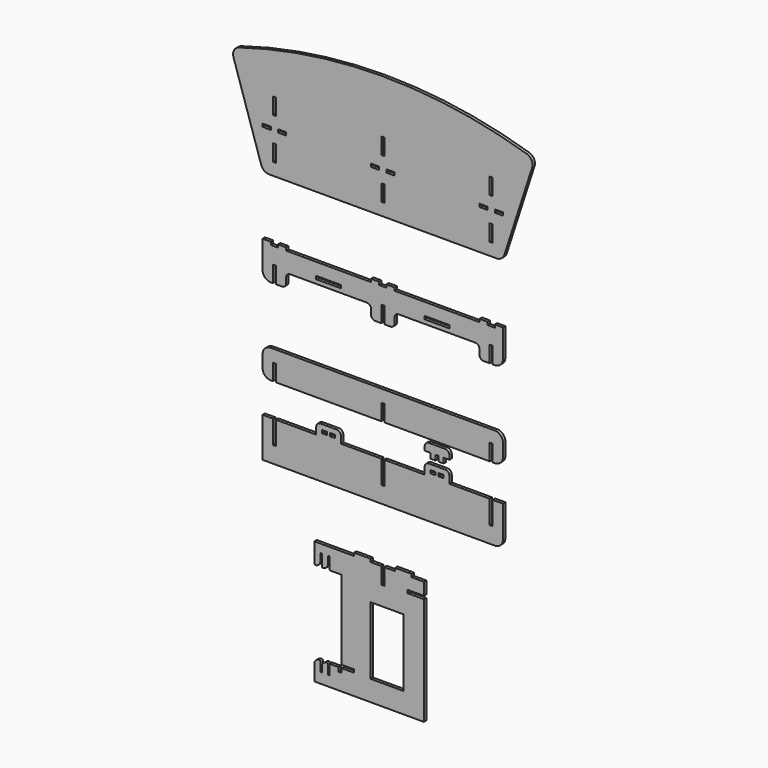
from build123d import *

# Parameters (mm, degrees)
F0_W     = 203.2
F0_H     = 417.195
F1_DEPTH = 18.542
F0_W_2   = 152.4
F0_H_2   = 18.542
F0_W_3   = 50.8
F0_H_3   = 18.034
F0_W_4   = 18.542
F0_H_4   = 101.6
F0_W_5   = 31.75
F0_H_5   = 31.75


# Not quite as in the source:
# - a feature names something its author has since deleted; it is built from what else it names


with BuildPart() as f1:
    # F0 (on Front) → F1 (new body)
    with BuildSketch(Plane.XZ):
        with BuildLine():
            Line((-177.8, 381), (-254, 381))
            Line((-254, 381), (-423.3333333333, 381))
            Line((-423.3333333333, 381), (-423.3333333333, 260.35))
            ThreePointArc((-423.3333333333, 260.35), (-421.4734613939, 255.8598719395), (-416.9833333333, 254))
            ThreePointArc((-416.9833333333, 254), (-394.5326930307, 263.2993596973), (-385.2333333333, 285.75))
            Line((-385.2333333333, 285.75), (-385.2333333333, 317.5))
            Line((-385.2333333333, 317.5), (-385.2333333333, 330.2))
            Line((-385.2333333333, 330.2), (-376.3433333333, 330.2))
            Line((-376.3433333333, 330.2), (-376.3433333333, 317.5))
            Line((-376.3433333333, 317.5), (-376.3433333333, 260.35))
            ThreePointArc((-376.3433333333, 260.35), (-374.4834613939, 255.8598719395), (-369.9933333333, 254))
            ThreePointArc((-369.9933333333, 254), (-347.5426930307, 263.2993596973), (-338.2433333333, 285.75))
            Line((-338.2433333333, 285.75), (-338.2433333333, 317.5))
            Line((-338.2433333333, 317.5), (-338.2433333333, 330.2))
            Line((-338.2433333333, 330.2), (-329.3533333333, 330.2))
            Line((-329.3533333333, 330.2), (-329.3533333333, 317.5))
            Line((-329.3533333333, 317.5), (-329.3533333333, 260.35))
            ThreePointArc((-329.3533333333, 260.35), (-327.4934613939, 255.8598719395), (-323.0033333333, 254))
            Line((-323.0033333333, 254), (-254, 254))
            Line((-254, 254), (-254, -235.458))
            Line((-254, -235.458), (-177.8, -235.458))
            Line((-177.8, -235.458), (-177.8, -254))
            Line((-177.8, -254), (-254, -254))
            Line((-254, -254), (-254, -279.4))
            Line((-254, -279.4), (-272.542, -279.4))
            Line((-272.542, -279.4), (-272.542, -254))
            Line((-272.542, -254), (-329.3533333333, -254))
            Line((-329.3533333333, -254), (-329.3533333333, -317.5))
            Line((-329.3533333333, -317.5), (-338.2433333333, -317.5))
            Line((-338.2433333333, -317.5), (-338.2433333333, -260.35))
            ThreePointArc((-338.2433333333, -260.35), (-340.1032052728, -255.8598719395), (-344.5933333333, -254))
            ThreePointArc((-344.5933333333, -254), (-367.043973636, -263.2993596973), (-376.3433333333, -285.75))
            Line((-376.3433333333, -285.75), (-376.3433333333, -317.5))
            Line((-376.3433333333, -317.5), (-385.2333333333, -317.5))
            Line((-385.2333333333, -317.5), (-385.2333333333, -260.35))
            ThreePointArc((-385.2333333333, -260.35), (-387.0932052728, -255.8598719395), (-391.5833333333, -254))
            ThreePointArc((-391.5833333333, -254), (-414.033973636, -263.2993596973), (-423.3333333333, -285.75))
            Line((-423.3333333333, -285.75), (-423.3333333333, -381))
            Line((-423.3333333333, -381), (-254, -381))
            Line((-254, -381), (254, -381))
            Line((254, -381), (254, 286.258))
            Line((254, 286.258), (152.4, 286.258))
            Line((152.4, 286.258), (152.4, 304.8))
            Line((152.4, 304.8), (254, 304.8))
            Line((254, 304.8), (254, 381))
            Line((254, 381), (177.8, 381))
            Line((177.8, 381), (177.8, 399.1356))
            Line((177.8, 399.1356), (76.2, 399.1356))
            Line((76.2, 399.1356), (76.2, 381))
            Line((76.2, 381), (9.0678, 381))
            Line((9.0678, 381), (9.0678, 279.4))
            Line((9.0678, 279.4), (-9.0678, 279.4))
            Line((-9.0678, 279.4), (-9.0678, 381))
            Line((-9.0678, 381), (-76.2, 381))
            Line((-76.2, 381), (-76.2, 399.1356))
            Line((-76.2, 399.1356), (-177.8, 399.1356))
            Line((-177.8, 399.1356), (-177.8, 381))
        make_face()
        with Locations((25.4, -45.4025)):
            Rectangle(F0_W, F0_H, mode=Mode.SUBTRACT)
    extrude(amount=F1_DEPTH)


with BuildPart() as f1b:
    # F0 (on Front) → F1, piece 2 (new body)
    with BuildSketch(Plane.XZ):
        with BuildLine():
            Line((691.945207411, 1346.2), (-691.945207411, 1346.2))
            ThreePointArc((-691.945207411, 1346.2), (-727.8662318953, 1331.3210244843), (-742.745207411, 1295.4))
            Line((-742.745207411, 1295.4), (-742.745207411, 1219.2))
            ThreePointArc((-742.745207411, 1219.2), (-727.8662318953, 1183.2789755157), (-691.945207411, 1168.4))
            Line((-691.945207411, 1168.4), (-679.245207411, 1168.4))
            Line((-679.245207411, 1168.4), (-679.245207411, 1270))
            Line((-679.245207411, 1270), (-660.703207411, 1270))
            Line((-660.703207411, 1270), (-660.703207411, 1168.4))
            Line((-660.703207411, 1168.4), (-9.271, 1168.4))
            Line((-9.271, 1168.4), (-9.271, 1270))
            Line((-9.271, 1270), (9.271, 1270))
            Line((9.271, 1270), (9.271, 1168.4))
            Line((9.271, 1168.4), (660.703207411, 1168.4))
            Line((660.703207411, 1168.4), (660.703207411, 1270))
            Line((660.703207411, 1270), (679.245207411, 1270))
            Line((679.245207411, 1270), (679.245207411, 1168.4))
            Line((679.245207411, 1168.4), (691.945207411, 1168.4))
            ThreePointArc((691.945207411, 1168.4), (727.8662318953, 1183.2789755157), (742.745207411, 1219.2))
            Line((742.745207411, 1219.2), (742.745207411, 1295.4))
            ThreePointArc((742.745207411, 1295.4), (727.8662318953, 1331.3210244843), (691.945207411, 1346.2))
        make_face()
    extrude(amount=F1_DEPTH)


with BuildPart() as f1c:
    # F0 (on Front) → F1, piece 3 (new body)
    with BuildSketch(Plane.XZ):
        with BuildLine():
            Line((-691.945207411, 1905), (-742.745207411, 1905))
            Line((-742.745207411, 1905), (-742.745207411, 1752.6))
            ThreePointArc((-742.745207411, 1752.6), (-727.8662318953, 1716.6789755157), (-691.945207411, 1701.8))
            Line((-691.945207411, 1701.8), (-679.245207411, 1701.8))
            Line((-679.245207411, 1701.8), (-679.245207411, 1803.4))
            Line((-679.245207411, 1803.4), (-660.703207411, 1803.4))
            Line((-660.703207411, 1803.4), (-660.703207411, 1701.8))
            Line((-660.703207411, 1701.8), (-622.603207411, 1701.8))
            ThreePointArc((-622.603207411, 1701.8), (-604.6426951688, 1709.2394877579), (-597.203207411, 1727.2))
            Line((-597.203207411, 1727.2), (-597.203207411, 1759.458))
            ThreePointArc((-597.203207411, 1759.458), (-589.7637196531, 1777.4185122421), (-571.803207411, 1784.858))
            Line((-571.803207411, 1784.858), (-98.171, 1784.858))
            ThreePointArc((-98.171, 1784.858), (-80.2104877579, 1777.4185122421), (-72.771, 1759.458))
            Line((-72.771, 1759.458), (-72.771, 1727.2))
            ThreePointArc((-72.771, 1727.2), (-65.3315122421, 1709.2394877579), (-47.371, 1701.8))
            Line((-47.371, 1701.8), (-9.271, 1701.8))
            Line((-9.271, 1701.8), (-9.271, 1803.4))
            Line((-9.271, 1803.4), (9.271, 1803.4))
            Line((9.271, 1803.4), (9.271, 1701.8))
            Line((9.271, 1701.8), (47.371, 1701.8))
            ThreePointArc((47.371, 1701.8), (65.3315122421, 1709.2394877579), (72.771, 1727.2))
            Line((72.771, 1727.2), (72.771, 1759.458))
            ThreePointArc((72.771, 1759.458), (80.2104877579, 1777.4185122421), (98.171, 1784.858))
            Line((98.171, 1784.858), (571.803207411, 1784.858))
            ThreePointArc((571.803207411, 1784.858), (589.7637196531, 1777.4185122421), (597.203207411, 1759.458))
            Line((597.203207411, 1759.458), (597.203207411, 1727.2))
            ThreePointArc((597.203207411, 1727.2), (604.6426951688, 1709.2394877579), (622.603207411, 1701.8))
            Line((622.603207411, 1701.8), (660.703207411, 1701.8))
            Line((660.703207411, 1701.8), (660.703207411, 1803.4))
            Line((660.703207411, 1803.4), (679.245207411, 1803.4))
            Line((679.245207411, 1803.4), (679.245207411, 1701.8))
            Line((679.245207411, 1701.8), (691.945207411, 1701.8))
            ThreePointArc((691.945207411, 1701.8), (727.8662318953, 1716.6789755157), (742.745207411, 1752.6))
            Line((742.745207411, 1752.6), (742.745207411, 1905))
            Line((742.745207411, 1905), (691.945207411, 1905))
            Line((691.945207411, 1905), (648.003207411, 1905))
            Line((648.003207411, 1905), (597.203207411, 1905))
            Line((597.203207411, 1905), (72.771, 1905))
            Line((72.771, 1905), (21.971, 1905))
            Line((21.971, 1905), (-21.971, 1905))
            Line((-21.971, 1905), (-72.771, 1905))
            Line((-72.771, 1905), (-597.203207411, 1905))
            Line((-597.203207411, 1905), (-648.003207411, 1905))
            Line((-648.003207411, 1905), (-691.945207411, 1905))
        make_face()
        with Locations((-334.9871037055, 1819.529)):
            Rectangle(F0_W_2, F0_H_2, mode=Mode.SUBTRACT)
        with Locations((334.9871037055, 1819.529)):
            Rectangle(F0_W_2, F0_H_2, mode=Mode.SUBTRACT)
        with Locations((-717.345207411, 1914.017)):
            Rectangle(F0_W_3, F0_H_3)
        with Locations((-622.603207411, 1914.017)):
            Rectangle(F0_W_3, F0_H_3)
        with Locations((-47.371, 1914.017)):
            Rectangle(F0_W_3, F0_H_3)
        with Locations((47.371, 1914.017)):
            Rectangle(F0_W_3, F0_H_3)
        with Locations((622.603207411, 1914.017)):
            Rectangle(F0_W_3, F0_H_3)
        with Locations((717.345207411, 1914.017)):
            Rectangle(F0_W_3, F0_H_3)
    extrude(amount=F1_DEPTH)


with BuildPart() as f1d:
    # F0 (on Front) → F1, piece 4 (new body)
    with BuildSketch(Plane.XZ):
        with BuildLine():
            ThreePointArc((0, 3048), (-449.4470794405, 3014.6809653399), (-889.0679496829, 2915.452311537))
            ThreePointArc((-889.0679496829, 2915.452311537), (-919.2876316446, 2890.361765082), (-922.5828932993, 2851.2221949528))
            Line((-922.5828932993, 2851.2221949528), (-751.0685099201, 2321.1607552747))
            ThreePointArc((-751.0685099201, 2321.1607552747), (-732.6202645277, 2295.7201166503), (-702.7357671423, 2286))
            Line((-702.7357671423, 2286), (0, 2286))
            Line((0, 2286), (702.7357671423, 2286))
            ThreePointArc((702.7357671423, 2286), (732.6202645277, 2295.7201166503), (751.0685099201, 2321.1607552747))
            Line((751.0685099201, 2321.1607552747), (922.5828932993, 2851.2221949528))
            ThreePointArc((922.5828932993, 2851.2221949528), (919.2876316446, 2890.361765082), (889.0679496829, 2915.452311537))
            ThreePointArc((889.0679496829, 2915.452311537), (449.4470794405, 3014.6809653399), (0, 3048))
        make_face()
        with Locations((-717.345207411, 2540.2032)):
            Rectangle(F0_W_3, F0_H_2, mode=Mode.SUBTRACT)
        with Locations((-669.974207411, 2413)):
            Rectangle(F0_W_4, F0_H_4, mode=Mode.SUBTRACT)
        with Locations((-622.603207411, 2540.2032)):
            Rectangle(F0_W_3, F0_H_2, mode=Mode.SUBTRACT)
        with Locations((-669.974207411, 2667.4064)):
            Rectangle(F0_W_4, F0_H_4, mode=Mode.SUBTRACT)
        with Locations((-47.371, 2540.2032)):
            Rectangle(F0_W_3, F0_H_2, mode=Mode.SUBTRACT)
        Polygon((9.271, 2362.2), (0, 2362.2), (-9.271, 2362.2), (-9.271, 2463.8), (9.271, 2463.8), align=None, mode=Mode.SUBTRACT)
        with Locations((47.371, 2540.2032)):
            Rectangle(F0_W_3, F0_H_2, mode=Mode.SUBTRACT)
        with Locations((0, 2667.4064)):
            Rectangle(F0_W_4, F0_H_4, mode=Mode.SUBTRACT)
        with Locations((669.974207411, 2413)):
            Rectangle(F0_W_4, F0_H_4, mode=Mode.SUBTRACT)
        with Locations((622.603207411, 2540.2032)):
            Rectangle(F0_W_3, F0_H_2, mode=Mode.SUBTRACT)
        with Locations((717.345207411, 2540.2032)):
            Rectangle(F0_W_3, F0_H_2, mode=Mode.SUBTRACT)
        with Locations((669.974207411, 2667.4064)):
            Rectangle(F0_W_4, F0_H_4, mode=Mode.SUBTRACT)
    extrude(amount=F1_DEPTH)


with BuildPart() as f1e:
    # F0 (on Front) → F1, piece 5 (new body)
    with BuildSketch(Plane.XZ):
        with BuildLine():
            Line((-411.1871037055, 1008.634), (-411.1871037055, 965.2))
            Line((-411.1871037055, 965.2), (-258.7871037055, 965.2))
            Line((-258.7871037055, 965.2), (-258.7871037055, 1008.634))
            ThreePointArc((-258.7871037055, 1008.634), (-266.2265914634, 1026.5945122421), (-284.1871037055, 1034.034))
            Line((-284.1871037055, 1034.034), (-385.7871037055, 1034.034))
            ThreePointArc((-385.7871037055, 1034.034), (-403.7476159476, 1026.5945122421), (-411.1871037055, 1008.634))
        make_face()
        with Locations((-360.1331037055, 993.013)):
            Rectangle(F0_W_5, F0_H_2, mode=Mode.SUBTRACT)
        with Locations((-309.8411037055, 993.013)):
            Rectangle(F0_W_5, F0_H_2, mode=Mode.SUBTRACT)
        Polygon((-411.1871037055, 965.2), (-660.703207411, 965.2), (-660.703207411, 821.8678), (-660.703207411, 720.2678), (-9.271, 720.2678), (-9.271, 821.8678), (-9.271, 965.2), (-258.7871037055, 965.2), align=None)
        Polygon((9.271, 821.8678), (9.271, 720.2678), (660.703207411, 720.2678), (660.703207411, 821.8678), (660.703207411, 965.2), (411.1871037055, 965.2), (258.7871037055, 965.2), (9.271, 965.2), align=None)
        with BuildLine():
            Line((258.7871037055, 1008.634), (258.7871037055, 965.2))
            Line((258.7871037055, 965.2), (411.1871037055, 965.2))
            Line((411.1871037055, 965.2), (411.1871037055, 1008.634))
            ThreePointArc((411.1871037055, 1008.634), (403.7476159476, 1026.5945122421), (385.7871037055, 1034.034))
            Line((385.7871037055, 1034.034), (284.1871037055, 1034.034))
            ThreePointArc((284.1871037055, 1034.034), (266.2265914634, 1026.5945122421), (258.7871037055, 1008.634))
        make_face()
        with Locations((309.8411037055, 993.013)):
            Rectangle(F0_W_5, F0_H_2, mode=Mode.SUBTRACT)
        with Locations((360.1331037055, 993.013)):
            Rectangle(F0_W_5, F0_H_2, mode=Mode.SUBTRACT)
        with BuildLine():
            Line((679.245207411, 821.8678), (679.245207411, 720.2678))
            Line((679.245207411, 720.2678), (691.945207411, 720.2678))
            ThreePointArc((691.945207411, 720.2678), (727.8662318953, 735.1467755157), (742.745207411, 771.0678))
            Line((742.745207411, 771.0678), (742.745207411, 965.2))
            Line((742.745207411, 965.2), (679.245207411, 965.2))
            Line((679.245207411, 965.2), (679.245207411, 821.8678))
        make_face()
        with Locations((669.974207411, 771.0678)):
            Rectangle(F0_W_4, F0_H_4)
        with Locations((0, 771.0678)):
            Rectangle(F0_W_4, F0_H_4)
        Polygon((-679.245207411, 965.2), (-742.745207411, 965.2), (-742.745207411, 720.2678), (-679.245207411, 720.2678), (-679.245207411, 821.8678), align=None)
        with Locations((-669.974207411, 771.0678)):
            Rectangle(F0_W_4, F0_H_4)
    extrude(amount=F1_DEPTH)


with BuildPart() as f1f:
    # F0 (on Front) → F1, piece 6 (new body)
    with BuildSketch(Plane.XZ):
        with BuildLine():
            Line((385.7871037055, 1146.4305265427), (284.1871037055, 1146.4305265427))
            ThreePointArc((284.1871037055, 1146.4305265427), (266.2265914634, 1138.9910387848), (258.7871037055, 1121.0305265427))
            Line((258.7871037055, 1121.0305265427), (258.7871037055, 1095.6305265427))
            Line((258.7871037055, 1095.6305265427), (293.9661037055, 1095.6305265427))
            Line((293.9661037055, 1095.6305265427), (325.7161037055, 1095.6305265427))
            Line((325.7161037055, 1095.6305265427), (344.2581037055, 1095.6305265427))
            Line((344.2581037055, 1095.6305265427), (376.0081037055, 1095.6305265427))
            Line((376.0081037055, 1095.6305265427), (411.1871037055, 1095.6305265427))
            Line((411.1871037055, 1095.6305265427), (411.1871037055, 1121.0305265427))
            ThreePointArc((411.1871037055, 1121.0305265427), (403.7476159476, 1138.9910387848), (385.7871037055, 1146.4305265427))
        make_face()
        with Locations((309.8411037055, 1079.7555265427)):
            Rectangle(F0_W_5, F0_H_5)
        with Locations((360.1331037055, 1079.7555265427)):
            Rectangle(F0_W_5, F0_H_5)
    extrude(amount=F1_DEPTH)


solid = Compound([f1.part, f1b.part, f1c.part, f1d.part, f1e.part, f1f.part])
